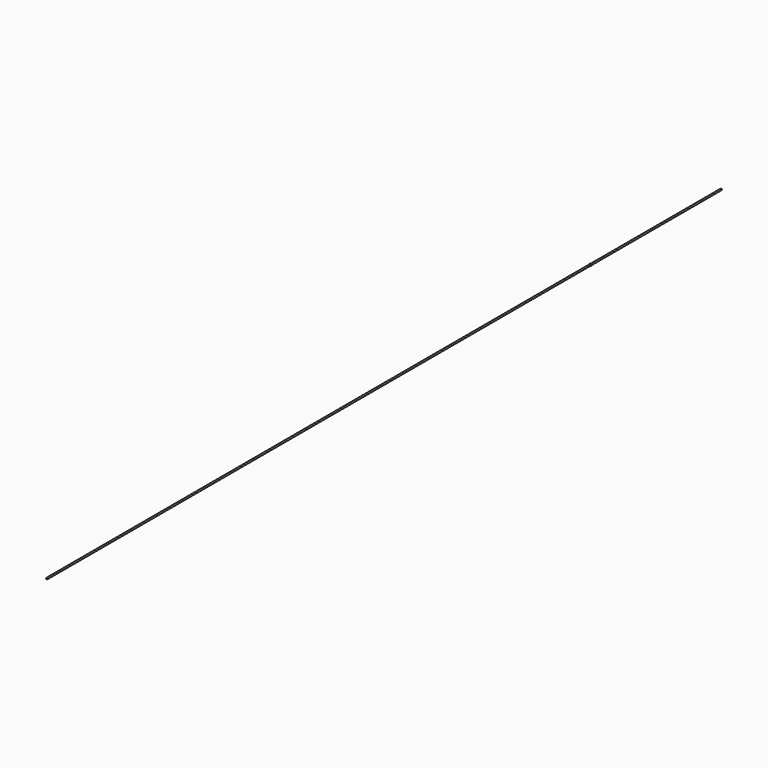
from build123d import *

# Parameters (mm, degrees)
F0_R        = 0.4445
F1_DEPTH    = 508
F3_R        = 0.635
F4_DEPTH    = 2.54
F5_S5_R     = 0.4445
F5_T6_DEPTH = 3
F6_S5_R     = 0.4445
F6_T6_DEPTH = 3
F7_R        = 0.4191


# Not quite as in the source:
# - a fillet or chamfer that OpenCascade refuses, or shapes differently, is made with other operations: its cross-section is extruded or revolved along the edge and cut away or added


with BuildPart() as f1:
    # F0 (on Front) → F1 (new body)
    with BuildSketch(Plane.XZ):
        Circle(F0_R)
    extrude(amount=F1_DEPTH)

    # F3 (on offset) → F4 (join)
    with BuildSketch(Plane.XZ.offset(99.822)):
        Circle(F3_R)
    extrude(amount=-F4_DEPTH)

    # F5: chamfer of 1.016 x 0.508 on 1 edges, made by hand


with BuildPart() as f5_tool2:
    # F5_s3 → F5_t4 (revolve)
    with BuildSketch(Plane.XY):
        Polygon((0.127, -97.282), (0.635, -98.298), (0.635, -97.282), align=None)
    revolve(axis=Axis((0, -97.282, 0), (0, -1, 0)))

    # F5_s5 → F5_t6 (cut, symmetric)
    with BuildSketch(Plane.XZ.offset(97.8)):
        Circle(F5_S5_R)
    extrude(amount=F5_T6_DEPTH, both=True, mode=Mode.SUBTRACT)


with BuildPart() as f1_1:
    add(f1.part)

    # F5_t1: cut F5_tool2
    add(f5_tool2.part, mode=Mode.SUBTRACT)

    # F6: chamfer of 0.508 x 1.016 on 1 edges, made by hand


with BuildPart() as f6_tool2:
    # F6_s3 → F6_t4 (revolve)
    with BuildSketch(Plane.XY):
        Polygon((0.635, -98.806), (0.127, -99.822), (0.635, -99.822), align=None)
    revolve(axis=Axis((0, -99.822, 0), (0, -1, 0)))

    # F6_s5 → F6_t6 (cut, symmetric)
    with BuildSketch(Plane.XZ.offset(99.3)):
        Circle(F6_S5_R)
    extrude(amount=F6_T6_DEPTH, both=True, mode=Mode.SUBTRACT)


with BuildPart() as f1_2:
    add(f1_1.part)

    # F6_t1: cut F6_tool2
    add(f6_tool2.part, mode=Mode.SUBTRACT)

    # F7
    f7_edges = [f1_2.edges().sort_by_distance(p)[0] for p in [
        (-0.4445, 0, 0),
    ]]
    fillet(f7_edges, radius=F7_R)


solid = f1_2.part
